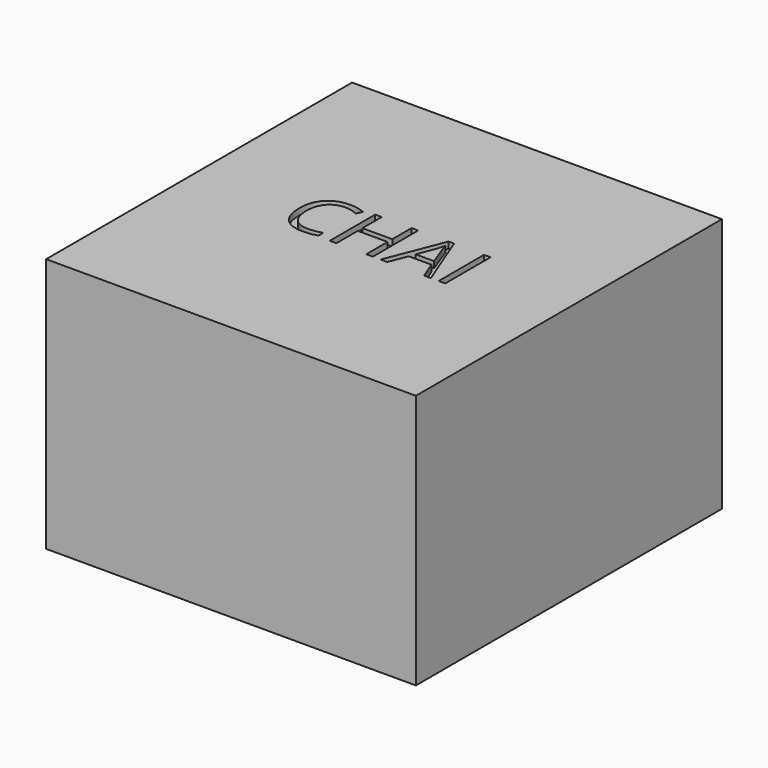
from build123d import *

# Parameters (mm, degrees)
F0_W         = 368.3
F0_H         = 381
F1_DEPTH     = 254
F2_TEXT_SIZE = 79.1101223582
F3_DEPTH     = 6.35


# Not quite as in the source:
# - Text() gives the source's letters only with a copy of the font that has no kerning and outlines rounded to 1/6400 em; it was checked with that copy


with BuildPart() as f1:
    # F0 (on Top) → F1 (new body)
    with BuildSketch(Plane.XY):
        with Locations((184.15, 190.5)):
            Rectangle(F0_W, F0_H)
    extrude(amount=F1_DEPTH)

    # F2 (on face) → F3 (cut)
    with BuildSketch(Plane.XY.offset(254)):
        with Locations((95.25, 162.0203559511)):
            Text('CHAI', F2_TEXT_SIZE, font='Open Sans', text_align=(TextAlign.LEFT, TextAlign.BOTTOM))
    extrude(amount=-F3_DEPTH, mode=Mode.SUBTRACT)


solid = f1.part
